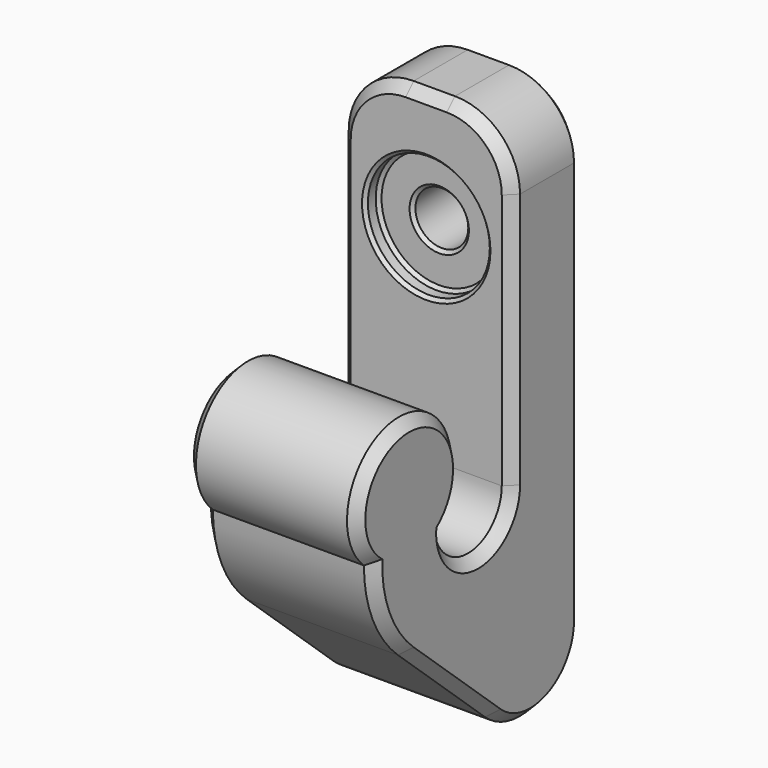
from build123d import *

# Parameters (mm, degrees)
F1_DEPTH   = 13.3858
F2_R       = 5.08
F3_R       = 2.06375
F4_DEPTH   = 25.4
F5_R       = 4.7625
F6_DEPTH   = 1.27
F7_C1_SIZE = 0.79375
F7_C2_SIZE = 0.79375
F7_C3_SIZE = 0.79365
F7_C4_SIZE = 0.79375
F8_SIZE    = 0.254


# Not quite as in the source:
# - a fillet or chamfer is up to 0.001 mm smaller than in the source, because OpenCascade refuses the exact size


with BuildPart() as f1:
    # F0 (on Right) → F1 (new body)
    with BuildSketch(Plane.YZ):
        with BuildLine():
            Line((10.16, -22.9468941689), (10.16, 25.0825))
            Line((10.16, 25.0825), (3.302, 25.0825))
            Line((3.302, 25.0825), (3.302, 0))
            ThreePointArc((3.302, 0), (0, -3.302), (-3.302, 0))
            ThreePointArc((-3.302, 0), (-6.731, 8.8281140591), (-10.16, 0))
            ThreePointArc((-10.16, 0), (-9.2901189355, -4.1133064758), (-6.8294310701, -7.5222650352))
            Line((-6.8294310701, -7.5222650352), (10.16, -22.9468941689))
        make_face()
    extrude(amount=F1_DEPTH)

    # F2
    f2_edges = [f1.edges().sort_by_distance(p)[0] for p in [
        (6.6929, 10.16, -22.946894),
        (13.3858, 6.731, 25.0825),
        (0, 6.731, 25.0825),
    ]]
    fillet(f2_edges, radius=F2_R)

    # F3 (on face) → F4 (cut)
    with BuildSketch(Plane.XZ.offset(-3.302)):
        with Locations((6.6929, 15.875)):
            Circle(F3_R)
    extrude(amount=-F4_DEPTH, mode=Mode.SUBTRACT)

    # F5 (on face) → F6 (cut)
    with BuildSketch(Plane.XZ.offset(-3.302)):
        with Locations((6.6929, 15.875)):
            Circle(F5_R)
    extrude(amount=-F6_DEPTH, mode=Mode.SUBTRACT)

    # F7: chamfer of 0.79375 on 16 edges, made by hand

    # F7_c1
    f7_c1_edges = [f1.edges().sort_by_distance(p)[0] for p in [
        (6.6929, 10.16, 25.0825),
        (1.4878975516, 10.16, 23.5946024484),
        (11.8979024484, 10.16, 23.5946024484),
        (0, 10.16, 4.2645264578),
        (13.3858, 10.16, 4.2645264578),
        (0, 7.1366532379, -16.1185065522),
        (0, -2.5820733026, -11.3784223186),
        (0, -9.2901189355, -4.1133064758),
        (13.3858, 7.1366532379, -16.1185065522),
        (13.3858, -2.5820733026, -11.3784223186),
        (13.3858, -9.2901189355, -4.1133064758),
    ]]
    chamfer(f7_c1_edges, length=F7_C1_SIZE)

    # F7_c2
    f7_c2_edges = [f1.edges().sort_by_distance(p)[0] for p in [
        (6.6929, 3.302, 25.0825),
        (1.4878975516, 3.302, 23.5946024484),
        (11.8979024484, 3.302, 23.5946024484),
        (0, 3.302, 10.00125),
        (0, 0, -3.302),
        (13.3858, 3.302, 10.00125),
        (13.3858, 0, -3.302),
    ]]
    chamfer(f7_c2_edges, length=F7_C2_SIZE)

    # F7_c3 (size 0.79375 in the source; OpenCascade refuses exactly that, so slightly less here)
    f7_c3_edges = [f1.edges().sort_by_distance(p)[0] for p in [
        (0, -6.731, 8.8281140591),
    ]]
    chamfer(f7_c3_edges, length=F7_C3_SIZE)

    # F7_c4
    f7_c4_edges = [f1.edges().sort_by_distance(p)[0] for p in [
        (13.3858, -6.731, 8.8281140591),
    ]]
    chamfer(f7_c4_edges, length=F7_C4_SIZE)

    # F8
    f8_edges = [f1.edges().sort_by_distance(p)[0] for p in [
        (11.4554, 3.937, 15.875),
        (1.9304, 3.302, 15.875),
        (1.9304, 4.572, 15.875),
        (4.62915, 4.572, 15.875),
        (8.75665, 7.366, 15.875),
        (4.62915, 10.16, 15.875),
    ]]
    chamfer(f8_edges, length=F8_SIZE)


solid = f1.part
